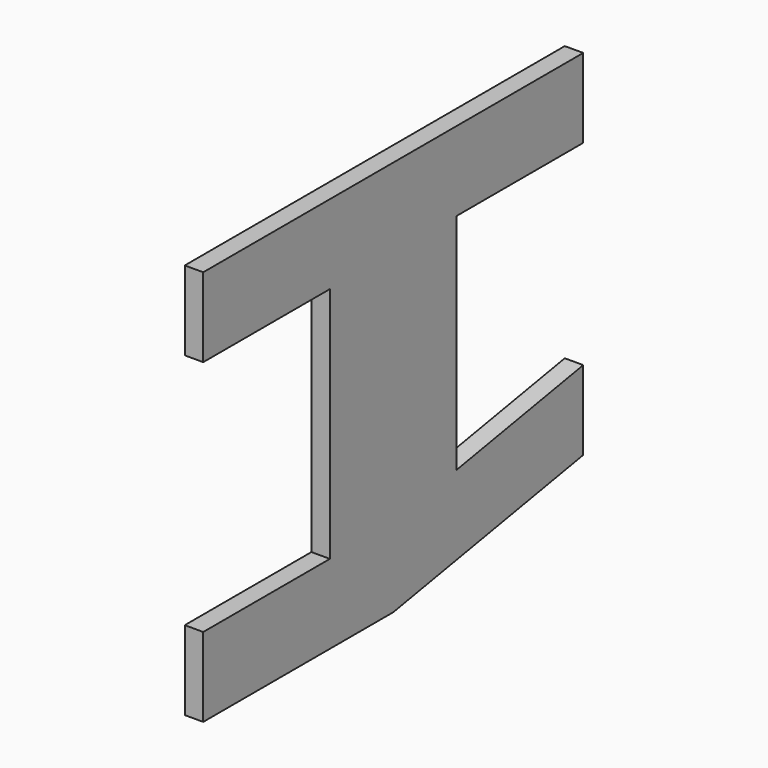
from build123d import *

# Parameters (mm, degrees)
F1_DEPTH = 7


# Not quite as in the source:
# - a feature names something its author has since deleted; it is built from what else it names


with BuildPart() as f1:
    # F0 (on Right) → F1 (new body)
    with BuildSketch(Plane.YZ):
        Polygon((-82.9850151411, 48.8100783943), (-22.9850151411, 48.8100783943), (-22.9850151411, -41.1170704361), (-22.9850151411, -41.1899216057), (-82.9850151411, -41.1899216057), (-82.9850151411, -71.1899216057), (7.0149848589, -71.1899216057), (97.0149848589, -55.320493342), (97.0149848589, -25.320493342), (37.0149848589, -35.9001121845), (37.0149848589, 48.8100783943), (97.0149848589, 48.8100783943), (97.0149848589, 78.8100783943), (7.0149848589, 78.8100783943), (-82.9850151411, 78.8100783943), align=None)
    extrude(amount=F1_DEPTH)


solid = f1.part
